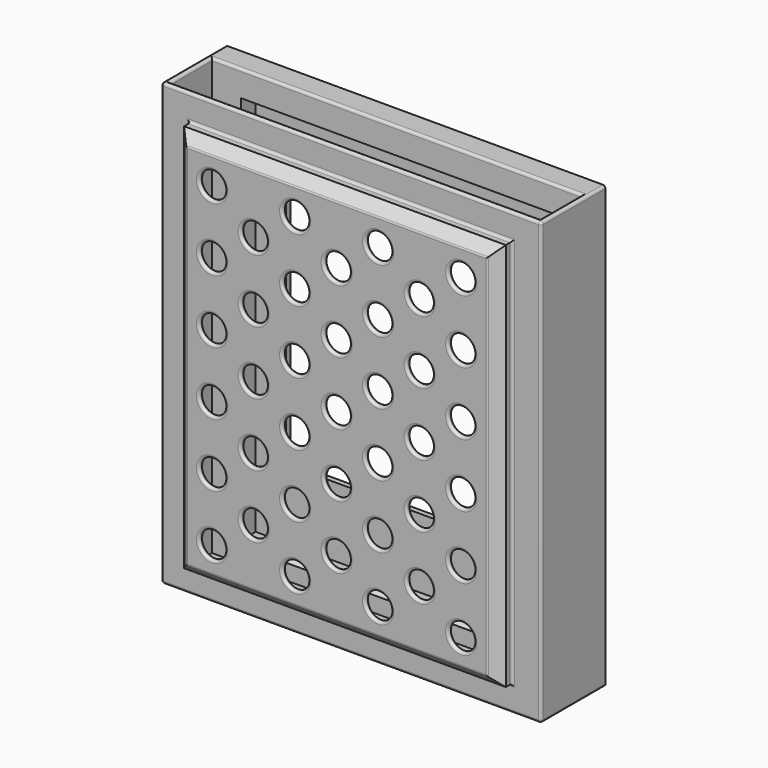
from build123d import *

# Parameters (mm, degrees)
F0_W      = 2.54
F0_H      = 2.54
F0_H_2    = 6.35
F0_W_2    = 11.7475
F0_W_3    = 152.4
F1_DEPTH  = 215.9
F2_W      = 122.555
F2_H      = 122.555
F3_DEPTH  = 2.54
F4_W      = 8.89
F4_H      = 2.54
F4_W_2    = 2.54
F4_W_3    = 25.4
F4_H_2    = 10.16
F4_H_3    = 12.7
F5_DEPTH  = 186.055
F6_W      = 8.89
F6_H      = 12.7
F7_DEPTH  = 157.48
F8_W      = 11.43
F8_H      = 2.54
F9_DEPTH  = 157.48
F10_SIZE  = 5.08
F11_R     = 1.26999
F12_SIZE  = 2.54
F13_R     = 6.35
F14_DEPTH = 2.54
F15_R     = 1.26999


# Not quite as in the source:
# - a fillet or chamfer is up to 0.001 mm smaller than in the source, because OpenCascade refuses the exact size
# - a feature names something its author has since deleted; it is built from what else it names


with BuildPart() as f1:
    # F0 (on Top) → F1 (new body)
    with BuildSketch(Plane.XY):
        with Locations((-91.7575, 44.45)):
            Rectangle(F0_W, F0_H)
        with Locations((-91.7575, 40.005)):
            Rectangle(F0_W, F0_H_2)
        with Locations((-84.61375, 44.45)):
            Rectangle(F0_W_2, F0_H)
        Polygon((-90.4875, 36.83), (-93.0275, 36.83), (-93.0275, 34.29), (-90.4875, 34.29), (-76.2, 34.29), (-76.2, 36.83), (-78.74, 36.83), align=None)
        with Locations((-77.47, 44.45)):
            Rectangle(F0_W, F0_H)
        Polygon((-90.4875, 34.29), (-93.0275, 34.29), (-93.0275, 6.35), (-90.4875, 6.35), (-90.4875, 8.89), align=None)
        with Locations((0, 44.45)):
            Rectangle(F0_W_3, F0_H)
        with Locations((77.47, 44.45)):
            Rectangle(F0_W, F0_H)
        Polygon((-76.2, 8.89), (-90.4875, 8.89), (-90.4875, 6.35), (-78.74, 6.35), (-76.2, 6.35), align=None)
        with Locations((84.61375, 44.45)):
            Rectangle(F0_W_2, F0_H)
        Polygon((-76.2, 6.35), (-78.74, 6.35), (-78.74, -2.54), (-76.2, -2.54), (-76.2, 0), align=None)
        Polygon((78.74, 36.83), (76.2, 36.83), (76.2, 34.29), (90.4875, 34.29), (93.0275, 34.29), (93.0275, 36.83), (90.4875, 36.83), align=None)
        with Locations((91.7575, 44.45)):
            Rectangle(F0_W, F0_H)
        with Locations((91.7575, 40.005)):
            Rectangle(F0_W, F0_H_2)
        with Locations((0, -1.27)):
            Rectangle(F0_W_3, F0_H)
        Polygon((93.0275, 34.29), (90.4875, 34.29), (90.4875, 8.89), (90.4875, 6.35), (93.0275, 6.35), align=None)
        Polygon((76.2, 6.35), (76.2, 0), (76.2, -2.54), (78.74, -2.54), (78.74, 6.35), align=None)
        Polygon((90.4875, 6.35), (90.4875, 8.89), (76.2, 8.89), (76.2, 6.35), (78.74, 6.35), align=None)
        with Locations((77.47, 40.005)):
            Rectangle(F0_W, F0_H_2)
        with Locations((-77.47, 40.005)):
            Rectangle(F0_W, F0_H_2)
    extrude(amount=F1_DEPTH)

    # F2 (on face) → F3 (cut, through all)
    with BuildSketch(Plane(origin=(0, 45.72, 0), x_dir=(-1, 0, 0), z_dir=(0, 1, 0))):
        with Locations((0, 107.95)):
            Rectangle(F2_W, F2_H)
    extrude(amount=-F3_DEPTH, mode=Mode.SUBTRACT)

    # F4 (on face) → F5 (join, through all)
    with BuildSketch(Plane(origin=(-93.0275, 0, 0), x_dir=(0, -1, 0), z_dir=(-1, 0, 0))):
        with Locations((-41.275, 214.63)):
            Rectangle(F4_W, F4_H)
        with Locations((-35.56, 214.63)):
            Rectangle(F4_W_2, F4_H)
        Polygon((-34.29, 213.36), (-36.83, 213.36), (-36.83, 205.74), (-36.83, 203.2), (-34.29, 203.2), align=None)
        with Locations((-41.275, 204.47)):
            Rectangle(F4_W, F4_H)
        with Locations((-41.275, 1.27)):
            Rectangle(F4_W, F4_H)
        with Locations((-35.56, 1.27)):
            Rectangle(F4_W_2, F4_H)
        with Locations((-21.59, 1.27)):
            Rectangle(F4_W_3, F4_H)
        Polygon((-36.83, 10.16), (-36.83, 2.54), (-34.29, 2.54), (-34.29, 12.7), (-36.83, 12.7), align=None)
        with Locations((-7.62, 1.27)):
            Rectangle(F4_W_2, F4_H)
        with Locations((-41.275, 11.43)):
            Rectangle(F4_W, F4_H)
        with Locations((-7.62, 7.62)):
            Rectangle(F4_W_2, F4_H_2)
        with Locations((-7.62, 209.55)):
            Rectangle(F4_W_2, F4_H_3)
    extrude(amount=-F5_DEPTH)

    # F6 (on face) → F7 (cut, through all)
    with BuildSketch(Plane.YZ.offset(78.74)):
        with Locations((1.905, 6.35)):
            Rectangle(F6_W, F6_H)
        with Locations((1.905, 209.55)):
            Rectangle(F6_W, F6_H)
    extrude(amount=-F7_DEPTH, mode=Mode.SUBTRACT)

    # F8 (on face) → F9 (join, through all)
    with BuildSketch(Plane.YZ.offset(78.74)):
        with Locations((3.175, 13.97)):
            Rectangle(F8_W, F8_H)
        with Locations((3.175, 201.93)):
            Rectangle(F8_W, F8_H)
    extrude(amount=-F9_DEPTH)

    # F10
    f10_edges = [f1.edges().sort_by_distance(p)[0] for p in [
        (0, -2.54, 203.2),
        (78.74, -2.54, 107.95),
        (-78.74, -2.54, 107.95),
        (0, -2.54, 12.7),
        (0, 0, 200.66),
        (-76.2, 0, 107.95),
        (0, 0, 15.24),
        (76.2, 0, 107.95),
    ]]
    chamfer(f10_edges, length=F10_SIZE)

    # F11 (radius 1.27 in the source; OpenCascade refuses exactly that, so slightly less here)
    f11_edges = [f1.edges().sort_by_distance(p)[0] for p in [
        (-93.0275, 6.35, 107.95),
        (0, 6.35, 215.9),
        (93.0275, 6.35, 107.95),
        (0, 6.35, 0),
        (-78.74, 6.35, 107.95),
        (0, 6.35, 12.7),
        (78.74, 6.35, 107.95),
        (0, 6.35, 203.2),
        (-93.0275, 26.035, 215.9),
        (-93.0275, 26.035, 0),
        (93.0275, 26.035, 215.9),
        (93.0275, 26.035, 0),
        (0, 34.29, 215.9),
        (0, 8.89, 215.9),
        (-90.4875, 21.59, 215.9),
        (90.4875, 21.59, 215.9),
    ]]
    fillet(f11_edges, radius=F11_R)

    # F12
    f12_edges = [f1.edges().sort_by_distance(p)[0] for p in [
        (0, 34.29, 12.7),
        (0, 8.89, 15.24),
    ]]
    chamfer(f12_edges, length=F12_SIZE)

    # F13 (on face) → F14 (cut, through all)
    with BuildSketch(Plane.XZ.offset(2.54)):
        with Locations((-60.96, 185.42)):
            Circle(F13_R)
        with Locations((-60.96, 154.432)):
            Circle(F13_R)
        with Locations((-60.96, 123.444)):
            Circle(F13_R)
        with Locations((-60.96, 92.456)):
            Circle(F13_R)
        with Locations((-60.96, 61.468)):
            Circle(F13_R)
        with Locations((-60.96, 30.48)):
            Circle(F13_R)
        with Locations((-20.32, 185.42)):
            Circle(F13_R)
        with Locations((-20.32, 154.432)):
            Circle(F13_R)
        with Locations((-20.32, 123.444)):
            Circle(F13_R)
        with Locations((-20.32, 92.456)):
            Circle(F13_R)
        with Locations((-20.32, 61.468)):
            Circle(F13_R)
        with Locations((-20.32, 30.48)):
            Circle(F13_R)
        with Locations((20.32, 185.42)):
            Circle(F13_R)
        with Locations((20.32, 154.432)):
            Circle(F13_R)
        with Locations((20.32, 123.444)):
            Circle(F13_R)
        with Locations((20.32, 92.456)):
            Circle(F13_R)
        with Locations((20.32, 61.468)):
            Circle(F13_R)
        with Locations((20.32, 30.48)):
            Circle(F13_R)
        with Locations((60.96, 185.42)):
            Circle(F13_R)
        with Locations((60.96, 154.432)):
            Circle(F13_R)
        with Locations((60.96, 123.444)):
            Circle(F13_R)
        with Locations((60.96, 92.456)):
            Circle(F13_R)
        with Locations((60.96, 61.468)):
            Circle(F13_R)
        with Locations((60.96, 30.48)):
            Circle(F13_R)
        with Locations((-40.64, 169.926)):
            Circle(F13_R)
        with Locations((-40.64, 138.938)):
            Circle(F13_R)
        with Locations((-40.64, 107.95)):
            Circle(F13_R)
        with Locations((-40.64, 76.962)):
            Circle(F13_R)
        with Locations((-40.64, 45.974)):
            Circle(F13_R)
        with Locations((0, 169.926)):
            Circle(F13_R)
        with Locations((0, 138.938)):
            Circle(F13_R)
        with Locations((0, 107.95)):
            Circle(F13_R)
        with Locations((0, 76.962)):
            Circle(F13_R)
        with Locations((0, 45.974)):
            Circle(F13_R)
        with Locations((40.64, 169.926)):
            Circle(F13_R)
        with Locations((40.64, 138.938)):
            Circle(F13_R)
        with Locations((40.64, 107.95)):
            Circle(F13_R)
        with Locations((40.64, 76.962)):
            Circle(F13_R)
        with Locations((40.64, 45.974)):
            Circle(F13_R)
    extrude(amount=-F14_DEPTH, mode=Mode.SUBTRACT)

    # F15 (radius 1.27 in the source; OpenCascade refuses exactly that, so slightly less here)
    f15_edges = [f1.edges().sort_by_distance(p)[0] for p in [
        (0, -2.54, 198.12),
        (73.66, -2.54, 107.95),
        (-73.66, -2.54, 107.95),
        (0, -2.54, 17.78),
        (-67.31, -2.54, 185.42),
        (-67.31, -2.54, 154.432),
        (-46.99, -2.54, 169.926),
        (-26.67, -2.54, 185.42),
        (-26.67, -2.54, 154.432),
        (-46.99, -2.54, 138.938),
        (-67.31, -2.54, 123.444),
        (-46.99, -2.54, 107.95),
        (-26.67, -2.54, 123.444),
        (13.97, -2.54, 185.42),
        (-6.35, -2.54, 169.926),
        (13.97, -2.54, 154.432),
        (54.61, -2.54, 185.42),
        (34.29, -2.54, 169.926),
        (54.61, -2.54, 154.432),
        (-6.35, -2.54, 138.938),
        (-6.35, -2.54, 107.95),
        (13.97, -2.54, 123.444),
        (34.29, -2.54, 138.938),
        (34.29, -2.54, 107.95),
        (54.61, -2.54, 123.444),
        (-67.31, -2.54, 92.456),
        (-46.99, -2.54, 76.962),
        (-26.67, -2.54, 92.456),
        (-67.31, -2.54, 61.468),
        (-46.99, -2.54, 45.974),
        (-67.31, -2.54, 30.48),
        (-26.67, -2.54, 61.468),
        (-26.67, -2.54, 30.48),
        (13.97, -2.54, 92.456),
        (-6.35, -2.54, 76.962),
        (54.61, -2.54, 92.456),
        (34.29, -2.54, 76.962),
        (-6.35, -2.54, 45.974),
        (13.97, -2.54, 61.468),
        (13.97, -2.54, 30.48),
        (34.29, -2.54, 45.974),
        (54.61, -2.54, 61.468),
        (54.61, -2.54, 30.48),
        (0, 0, 195.58),
        (-71.12, 0, 107.95),
        (71.12, 0, 107.95),
        (0, 0, 20.32),
        (54.61, 0, 185.42),
        (54.61, 0, 154.432),
        (34.29, 0, 169.926),
        (13.97, 0, 185.42),
        (13.97, 0, 154.432),
        (34.29, 0, 138.938),
        (54.61, 0, 123.444),
        (34.29, 0, 107.95),
        (13.97, 0, 123.444),
        (-26.67, 0, 185.42),
        (-6.35, 0, 169.926),
        (-26.67, 0, 154.432),
        (-67.31, 0, 185.42),
        (-46.99, 0, 169.926),
        (-67.31, 0, 154.432),
        (-6.35, 0, 138.938),
        (-6.35, 0, 107.95),
        (-26.67, 0, 123.444),
        (-46.99, 0, 138.938),
        (-46.99, 0, 107.95),
        (-67.31, 0, 123.444),
        (54.61, 0, 92.456),
        (34.29, 0, 76.962),
        (13.97, 0, 92.456),
        (54.61, 0, 61.468),
        (34.29, 0, 45.974),
        (54.61, 0, 30.48),
        (13.97, 0, 61.468),
        (13.97, 0, 30.48),
        (-26.67, 0, 92.456),
        (-6.35, 0, 76.962),
        (-67.31, 0, 92.456),
        (-46.99, 0, 76.962),
        (-6.35, 0, 45.974),
        (-26.67, 0, 61.468),
        (-26.67, 0, 30.48),
        (-46.99, 0, 45.974),
        (-67.31, 0, 61.468),
        (-67.31, 0, 30.48),
    ]]
    fillet(f15_edges, radius=F15_R)


solid = f1.part
